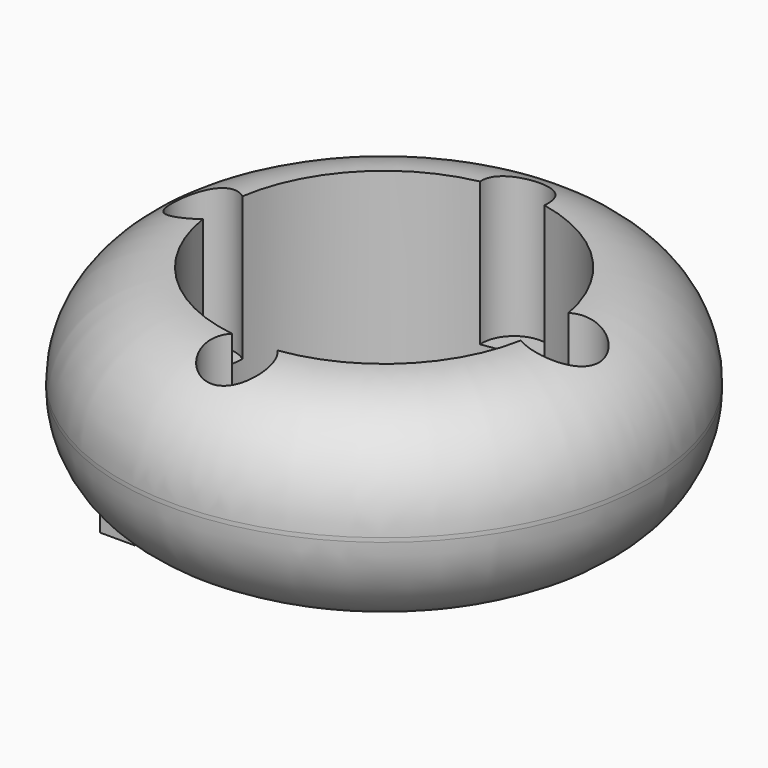
from build123d import *

# Parameters (mm, degrees)
F0_R         = 65.9510645132
F1_DEPTH     = 51.308
F2_R         = 25.1416200386
F4_DEPTH     = 45.72
F5_R         = 8.076157776
F5_R_2       = 8.7943033274
F5_R_3       = 7.9415704541
F5_R_4       = 7.8322177361
F6_DEPTH     = 61.214
F7_TEXT_SIZE = 28.2060380818
F8_DEPTH     = 9.652


# Not quite as in the source:
# - Text() gives the source's letters only with a copy of the font that has no kerning and outlines rounded to 1/6400 em; it was checked with that copy


with BuildPart() as f1:
    # F0 (on Top) → F1 (new body)
    with BuildSketch(Plane.XY):
        Circle(F0_R)
    extrude(amount=F1_DEPTH)

    # F2
    f2_edges = [f1.edges().sort_by_distance(p)[0] for p in [
        (-65.951065, 0, 51.308),
        (-65.951065, 0, 0),
    ]]
    fillet(f2_edges, radius=F2_R)

    # F4 (cut): a face of the model
    f4_faces = [f1.faces().sort_by_distance(p)[0] for p in [
        (0, 0, 51.308),
    ]]
    extrude(f4_faces, amount=-F4_DEPTH, mode=Mode.SUBTRACT)

    # F5 (on offset) → F6 (cut)
    with BuildSketch(Plane.XY.offset(76.708)):
        with Locations((0, 40.591981262)):
            Circle(F5_R)
        with Locations((44.8302254081, 0)):
            Circle(F5_R_2)
        with Locations((0, -45.9915697575)):
            Circle(F5_R_3)
        with Locations((-45.1435782015, 0)):
            Circle(F5_R_4)
    extrude(amount=-F6_DEPTH, mode=Mode.SUBTRACT)

    # F7 (on Top) → F8 (join)
    with BuildSketch(Plane.XY):
        with Locations((-46.3666506112, -30.7072009891)):
            Text('RKJ', F7_TEXT_SIZE, font='Tinos', font_style=FontStyle.BOLDITALIC, text_align=(TextAlign.LEFT, TextAlign.BOTTOM))
    extrude(amount=-F8_DEPTH)


solid = f1.part
